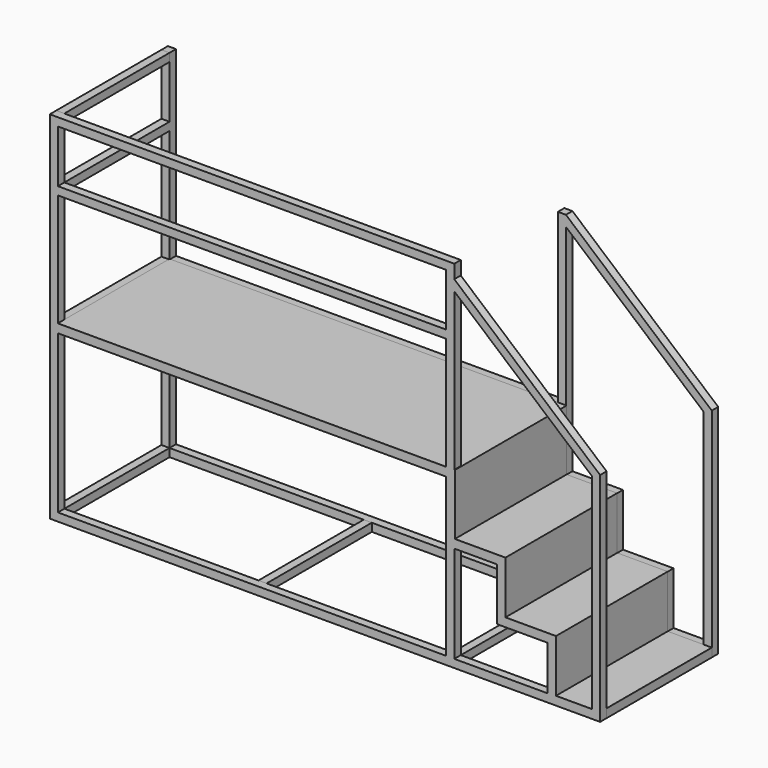
from build123d import *

# Parameters (mm, degrees)
F0_W      = 1920
F0_H      = 780
F0_H_2    = 860
F1_DEPTH  = 40
F2_W      = 40
F2_H      = 40
F3_DEPTH  = 650
F6_W      = 1920
F6_H      = 3
F6_W_2    = 40
F7_DEPTH  = 690
F9_DEPTH  = 760
F10_W     = 1920
F10_H     = 40
F11_DEPTH = 40
F12_W     = 664.210498333
F12_H     = 40
F13_DEPTH = 40


with BuildPart() as f1:
    # F0 (on Front) → F1 (new body)
    with BuildSketch(Plane.XZ):
        Polygon((0, -820), (2000, -820), (2720.8986186981, -820), (2720.8986186981, 254.5713696399), (2000, 872.3691137475), (2000, 940), (0, 940), (0, 40), (0, 0), align=None)
        with Locations((1000, -390)):
            Rectangle(F0_W, F0_H, mode=Mode.SUBTRACT)
        Polygon((2460, -780), (2000, -780), (2000, -300), (2210, -300), (2210, -560), (2460, -560), align=None, mode=Mode.SUBTRACT)
        Polygon((2000, 0), (2000, 40), (2000, 819.6901679039), (2680.8986186981, 236.1717373133), (2680.8986186981, -780), (2500, -780), (2500, -520), (2250, -520), (2250, -260), (2000, -260), align=None, mode=Mode.SUBTRACT)
        with Locations((1000, 470)):
            Rectangle(F0_W, F0_H_2, mode=Mode.SUBTRACT)
    extrude(amount=F1_DEPTH)


with BuildPart() as f3:
    # F2 (on face) → F3 (new body)
    with BuildSketch(Plane(origin=(0, 0, 0), x_dir=(-1, 0, 0), z_dir=(0, 1, 0))):
        with Locations((-20, 920)):
            Rectangle(F2_W, F2_H)
    extrude(amount=F3_DEPTH)


with BuildPart() as f3b:
    # F2 (on face) → F3, piece 2 (new body)
    with BuildSketch(Plane(origin=(0, 0, 0), x_dir=(-1, 0, 0), z_dir=(0, 1, 0))):
        with Locations((-20, 20)):
            Rectangle(F2_W, F2_H)
    extrude(amount=F3_DEPTH)


with BuildPart() as f3c:
    # F2 (on face) → F3, piece 3 (new body)
    with BuildSketch(Plane(origin=(0, 0, 0), x_dir=(-1, 0, 0), z_dir=(0, 1, 0))):
        with Locations((-20, -800)):
            Rectangle(F2_W, F2_H)
    extrude(amount=F3_DEPTH)


with BuildPart() as f3d:
    # F2 (on face) → F3, piece 4 (new body)
    with BuildSketch(Plane(origin=(0, 0, 0), x_dir=(-1, 0, 0), z_dir=(0, 1, 0))):
        with Locations((-1020, -800)):
            Rectangle(F2_W, F2_H)
    extrude(amount=F3_DEPTH)


with BuildPart() as f3e:
    # F2 (on face) → F3, piece 5 (new body)
    with BuildSketch(Plane(origin=(0, 0, 0), x_dir=(-1, 0, 0), z_dir=(0, 1, 0))):
        with Locations((-1020, 20)):
            Rectangle(F2_W, F2_H)
    extrude(amount=F3_DEPTH)


with BuildPart() as f3f:
    # F2 (on face) → F3, piece 6 (new body)
    with BuildSketch(Plane(origin=(0, 0, 0), x_dir=(-1, 0, 0), z_dir=(0, 1, 0))):
        with Locations((-1980, 20)):
            Rectangle(F2_W, F2_H)
    extrude(amount=F3_DEPTH)


with BuildPart() as f3g:
    # F2 (on face) → F3, piece 7 (new body)
    with BuildSketch(Plane(origin=(0, 0, 0), x_dir=(-1, 0, 0), z_dir=(0, 1, 0))):
        with Locations((-1980, -800)):
            Rectangle(F2_W, F2_H)
    extrude(amount=F3_DEPTH)


with BuildPart() as f3h:
    # F2 (on face) → F3, piece 8 (new body)
    with BuildSketch(Plane(origin=(0, 0, 0), x_dir=(-1, 0, 0), z_dir=(0, 1, 0))):
        with Locations((-1980, -280)):
            Rectangle(F2_W, F2_H)
    extrude(amount=F3_DEPTH)


with BuildPart() as f3i:
    # F2 (on face) → F3, piece 9 (new body)
    with BuildSketch(Plane(origin=(0, 0, 0), x_dir=(-1, 0, 0), z_dir=(0, 1, 0))):
        with Locations((-2230, -280)):
            Rectangle(F2_W, F2_H)
    extrude(amount=F3_DEPTH)


with BuildPart() as f3j:
    # F2 (on face) → F3, piece 10 (new body)
    with BuildSketch(Plane(origin=(0, 0, 0), x_dir=(-1, 0, 0), z_dir=(0, 1, 0))):
        with Locations((-2480, -540)):
            Rectangle(F2_W, F2_H)
    extrude(amount=F3_DEPTH)


with BuildPart() as f3k:
    # F2 (on face) → F3, piece 11 (new body)
    with BuildSketch(Plane(origin=(0, 0, 0), x_dir=(-1, 0, 0), z_dir=(0, 1, 0))):
        with Locations((-2230, -540)):
            Rectangle(F2_W, F2_H)
    extrude(amount=F3_DEPTH)


with BuildPart() as f3l:
    # F2 (on face) → F3, piece 12 (new body)
    with BuildSketch(Plane(origin=(0, 0, 0), x_dir=(-1, 0, 0), z_dir=(0, 1, 0))):
        with Locations((-2480, -800)):
            Rectangle(F2_W, F2_H)
    extrude(amount=F3_DEPTH)


with BuildPart() as f3m:
    # F2 (on face) → F3, piece 13 (new body)
    with BuildSketch(Plane(origin=(0, 0, 0), x_dir=(-1, 0, 0), z_dir=(0, 1, 0))):
        with Locations((-2700.8986186981, -800)):
            Rectangle(F2_W, F2_H)
    extrude(amount=F3_DEPTH)


with BuildPart() as f5_1:
    # F5: instance of F1
    add(f1.part.mirror(Plane(origin=(1405.4269340263, 325, -25.6106012705), x_dir=(1, 0, 0), z_dir=(0, 1, 0))))

    # F8 (on face) → F9 (cut)
    with BuildSketch(Plane(origin=(0, 690, 0), x_dir=(-1, 0, 0), z_dir=(0, 1, 0))):
        Polygon((-40, 940), (-2000, 940), (-2000, 872.3691137475), (-1960, 872.3691137475), (-1960, 900), (-40, 900), align=None)
    extrude(amount=-F9_DEPTH, mode=Mode.SUBTRACT)


with BuildPart() as f7:
    # F6 (on face) → F7 (new body)
    with BuildSketch(Plane.XZ.offset(40)):
        with Locations((1000, 41.5)):
            Rectangle(F6_W, F6_H)
        with Locations((1980, 41.5)):
            Rectangle(F6_W_2, F6_H)
        Polygon((2000, 43), (2000, 40), (2000, -260), (2250, -260), (2250, -520), (2500, -520), (2500, -780), (2680.8986186981, -780), (2680.8986186981, -777), (2503, -777), (2503, -517), (2253, -517), (2253, -257), (2003, -257), (2003, 43), align=None)
        with Locations((2700.8986186981, -778.5)):
            Rectangle(F6_W_2, F6_H)
    extrude(amount=-F7_DEPTH)


with BuildPart() as f1_1:
    add(f1.part)

    # F10 (on face) → F11 (join)
    with BuildSketch(Plane.XZ.offset(40)):
        with Locations((1000, 620)):
            Rectangle(F10_W, F10_H)
    extrude(amount=-F11_DEPTH)

    add(f5_1.part)  # F13 merges F5_1
    # F12 (on face) → F13 (join)
    with BuildSketch(Plane(origin=(0, 0, 0), x_dir=(0, -1, 0), z_dir=(-1, 0, 0))):
        with Locations((-332.1052491665, 620)):
            Rectangle(F12_W, F12_H)
    extrude(amount=-F13_DEPTH)


solid = Compound([f3.part, f3b.part, f3c.part, f3d.part, f3e.part, f3f.part, f3g.part, f3h.part, f3i.part, f3j.part, f3k.part, f3l.part, f3m.part, f7.part, f1_1.part])
